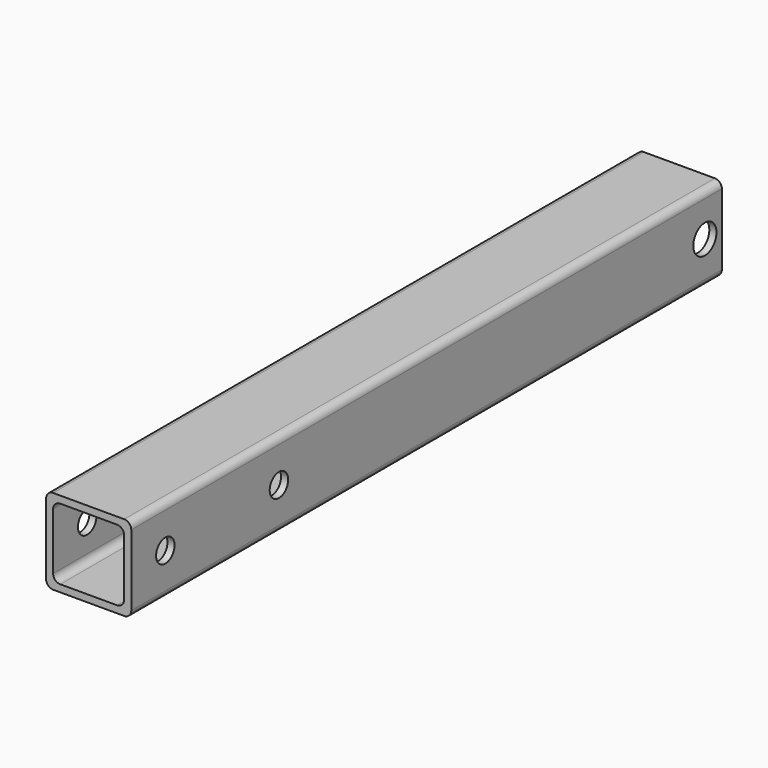
from build123d import *

# Parameters (mm, degrees)
F0_W     = 19.05
F0_H     = 19.05
F0_W_2   = 15.875
F0_H_2   = 15.875
F1_DEPTH = 107.95
F2_R     = 1.5875
F3_R     = 1.5875
F4_R     = 3.2385
F4_R_2   = 2.5796875
F5_DEPTH = 19.05
F6_DEPTH = 47.625
F7_DEPTH = 3.175


# Not quite as in the source:
# - a length typed as a fraction of an inch, garbled in the dataset ("3 / 203.2 mm" for 3/8 in), is restored


with BuildPart() as f1:
    # F0 (on Front) → F1 (new body, symmetric)
    with BuildSketch(Plane.XZ):
        Rectangle(F0_W, F0_H)
        with Locations((-0.0127, 0)):
            Rectangle(F0_W_2, F0_H_2, mode=Mode.SUBTRACT)
    extrude(amount=F1_DEPTH, both=True)

    # F2
    f2_edges = [f1.edges().sort_by_distance(p)[0] for p in [
        (-9.525, 0, 9.525),
        (-9.525, 0, -9.525),
        (9.525, 0, -9.525),
        (9.525, 0, 9.525),
    ]]
    fillet(f2_edges, radius=F2_R)

    # F3
    f3_edges = [f1.edges().sort_by_distance(p)[0] for p in [
        (-7.9502, 0, 7.9375),
        (-7.9502, 0, -7.9375),
        (7.9248, 0, 7.9375),
        (7.9248, 0, -7.9375),
    ]]
    fillet(f3_edges, radius=F3_R)

    # F4 (on face) → F5 (cut)
    with BuildSketch(Plane(origin=(-9.525, 0, 0), x_dir=(0, -1, 0), z_dir=(-1, 0, 0))):
        with Locations((-100.0125, 0)):
            Circle(F4_R)
        with Locations((19.05, 0)):
            Circle(F4_R_2)
        with Locations((50.8, 0)):
            Circle(F4_R_2)
    extrude(amount=-F5_DEPTH, mode=Mode.SUBTRACT)

    # F6 (cut): a face of the model
    f6_faces = [f1.faces().sort_by_distance(p)[0] for p in [
        (-8.2196076836, -107.95, 0),
    ]]
    extrude(f6_faces, amount=-F6_DEPTH, mode=Mode.SUBTRACT)

    # F7 (cut): a face of the model
    f7_faces = [f1.faces().sort_by_distance(p)[0] for p in [
        (-8.2196076836, 107.95, 0),
    ]]
    extrude(f7_faces, amount=-F7_DEPTH, mode=Mode.SUBTRACT)


solid = f1.part
